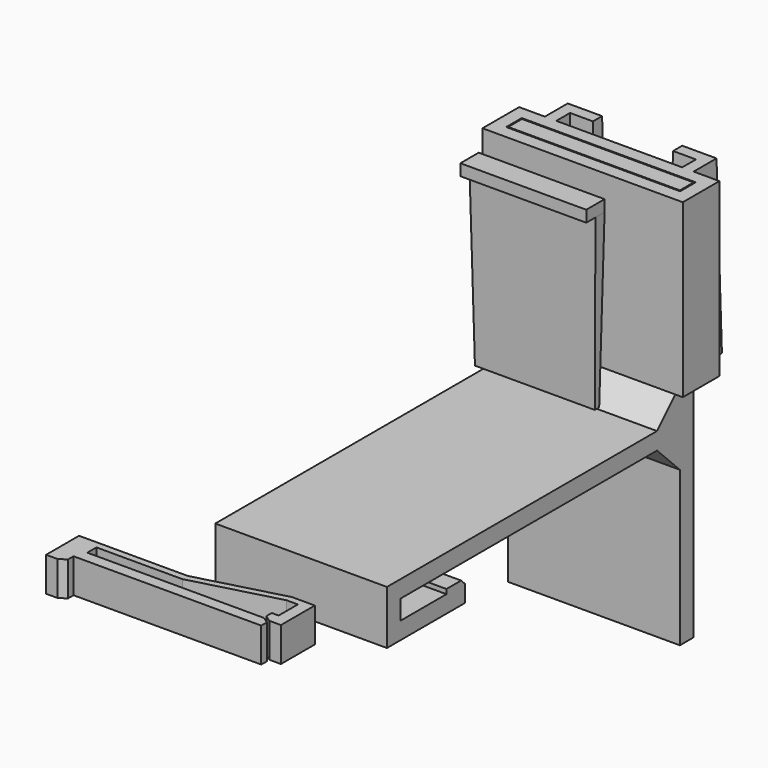
from build123d import *

# Parameters (mm, degrees)
F0_W      = 5
F0_H      = 5
F0_W_2    = 4
F0_H_2    = 0.8
F1_DEPTH  = 30
F3_W      = 30.4
F3_H      = 3.4
F4_DEPTH  = 30
F5_SIZE   = 0.8
F6_SIZE   = 4.99999
F3_W_2    = 22
F3_H_2    = 2
F7_DEPTH  = 30
F7_TAPER  = 1
F8_DEPTH  = 2
F9_W      = 30
F9_H      = 2
F9_W_2    = 15
F9_H_2    = 1.2
F9_W_3    = 2
F10_DEPTH = 6
F3_W_3    = 2
F3_H_3    = 3
F11_DEPTH = 30
F11_TAPER = -1


# Not quite as in the source:
# - a fillet or chamfer is up to 0.001 mm smaller than in the source, because OpenCascade refuses the exact size
# - a feature names something its author has since deleted; it is built from what else it names


with BuildPart() as f1:
    # F0 (on Right) → F1 (new body)
    with BuildSketch(Plane.YZ):
        Polygon((59, 0), (0, 0), (0, -3), (3, -3), (59, -3), (64, -3), (64, 0), align=None)
        with Locations((61.5, 2.5)):
            Rectangle(F0_W, F0_H)
        Polygon((3, -3), (0, -3), (0, -9.4), (3, -9.4), (3, -6.4), align=None)
        Polygon((67, 0), (64, 0), (64, -3), (64, -8), (64, -35), (67, -35), align=None)
        Polygon((64, 5), (64, 0), (67, 0), (67, 35), (64, 35), align=None)
        with Locations((61.5, -5.5)):
            Rectangle(F0_W, F0_H)
        Polygon((13, -6.4), (3, -6.4), (3, -9.4), (17, -9.4), (17, -6.4), align=None)
        with Locations((15, -6)):
            Rectangle(F0_W_2, F0_H_2)
    extrude(amount=F1_DEPTH)

    # F5
    f5_edges = [f1.edges().sort_by_distance(p)[0] for p in [
        (15, 17, -5.6),
    ]]
    chamfer(f5_edges, length=F5_SIZE)

    # F6 (size 5 in the source; OpenCascade refuses exactly that, so slightly less here)
    f6_edges = [f1.edges().sort_by_distance(p)[0] for p in [
        (15, 59, 5),
        (15, 59, -8),
    ]]
    chamfer(f6_edges, length=F6_SIZE)


with BuildPart() as f4:
    # F3 (on offset) → F4 (new body)
    with BuildSketch(Plane.XY.offset(35)):
        Polygon((2, 69.5), (-2.5, 69.5), (-2.5, 61.5), (32.5, 61.5), (32.5, 69.5), (28, 69.5), (28, 68.5), (2, 68.5), align=None)
        with Locations((15, 65.5)):
            Rectangle(F3_W, F3_H, mode=Mode.SUBTRACT)
        Polygon((4, 69.5), (2, 69.5), (2, 68.5), (28, 68.5), (28, 69.5), (26, 69.5), align=None)
    extrude(amount=-F4_DEPTH)

    # F3 (on offset) → F11 (join)
    with BuildSketch(Plane.XY.offset(35)):
        Polygon((22, 72.5), (26, 72.5), (28, 72.5), (28, 74.5), (22, 74.5), align=None)
        with Locations((27, 71)):
            Rectangle(F3_W_3, F3_H_3)
        Polygon((4, 69.5), (2, 69.5), (2, 68.5), (28, 68.5), (28, 69.5), (26, 69.5), align=None)
        Polygon((2, 74.5), (2, 72.5), (4, 72.5), (8, 72.5), (8, 74.5), align=None)
        with Locations((3, 71)):
            Rectangle(F3_W_3, F3_H_3)
    extrude(amount=-F11_DEPTH, taper=F11_TAPER)


with BuildPart() as f7:
    # F3 (on offset) → F7 (new body)
    with BuildSketch(Plane.XY.offset(35)):
        with Locations((15, 51.545239985)):
            Rectangle(F3_W_2, F3_H_2)
    extrude(amount=-F7_DEPTH, taper=F7_TAPER)

    # F3 (on offset) → F8 (join)
    with BuildSketch(Plane.XY.offset(35)):
        with Locations((15, 49.545239985)):
            Rectangle(F3_W_2, F3_H_2)
        with Locations((15, 51.545239985)):
            Rectangle(F3_W_2, F3_H_2)
    extrude(amount=F8_DEPTH)


with BuildPart() as f10:
    # F9 (on Top) → F10 (new body)
    with BuildSketch(Plane.XY):
        with Locations((13.9398306429, -27.6358266532)):
            Rectangle(F9_W, F9_H)
        Polygon((-1.0601693571, -28.6358266532), (-1.0601693571, -26.6358266532), (-1.0601693571, -24.6358266532), (-1.0601693571, -23.4358266532), (-5.0601693571, -23.4358266532), (-5.0601693571, -28.6358266532), (-3.0601693571, -28.6358266532), (-1.8601693571, -28.6358266532), align=None)
        with Locations((6.4398306429, -24.0358266532)):
            Rectangle(F9_W_2, F9_H_2)
        Polygon((13.9398306429, -23.4358266532), (13.9398306429, -24.6358266532), (28.9398306429, -20.6358266532), (28.9398306429, -19.4358266532), align=None)
        Polygon((29.8163002714, -26.6358266532), (28.9398306429, -26.6358266532), (28.9398306429, -28.6358266532), (30.9398306429, -28.6358266532), (30.9398306429, -27.3848469009), align=None)
        Polygon((28.9398306429, -19.4358266532), (28.9398306429, -20.6358266532), (30.9398306429, -20.6358266532), (32.9398306429, -20.6358266532), (32.9398306429, -19.4358266532), align=None)
        Polygon((30.9398306429, -24.8358266532), (30.9398306429, -26.6358266532), (30.9398306429, -26.8358266532), (32.9398306429, -26.8358266532), (32.9398306429, -20.6358266532), (30.9398306429, -20.6358266532), align=None)
        Polygon((29.7398306429, -26.0358266532), (30.6398306429, -26.6358266532), (30.9398306429, -26.6358266532), (30.9398306429, -24.8358266532), (29.7398306429, -24.8358266532), align=None)
        with Locations((-4.0601693571, -29.6358266532)):
            Rectangle(F9_W_3, F9_H)
        Polygon((-1.8601693571, -29.8358266532), (-1.8601693571, -28.6358266532), (-3.0601693571, -28.6358266532), (-3.0601693571, -30.6358266532), align=None)
        Polygon((30.9398306429, -26.6358266532), (30.6398306429, -26.6358266532), (30.9398306429, -26.8358266532), align=None)
    extrude(amount=F10_DEPTH)


solid = Compound([f1.part, f4.part, f7.part, f10.part])
